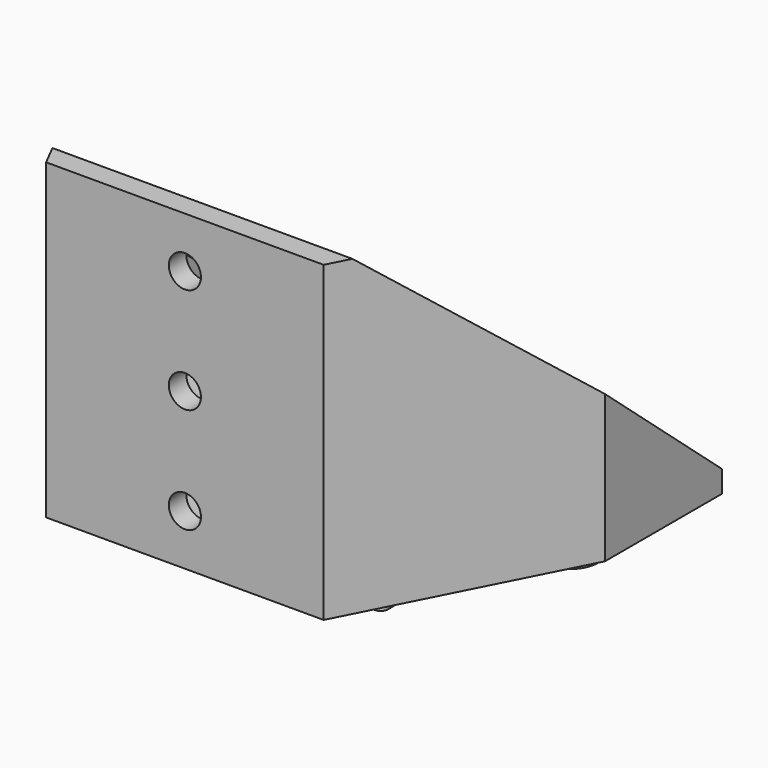
from build123d import *

# Parameters (mm, degrees)
F4_DEPTH       = 21.4
F5_DEPTH       = 1.5
F1_R           = 1.9
F1_W           = 19
F1_H           = 1.5
F6_DEPTH       = 1.6
F8_DEPTH       = 17.001
F8_DEPTH_BACK  = 17.001
F9_R           = 1.15
F10_DEPTH      = 21.401
F10_DEPTH_BACK = 1.601
F11_R          = 1.1
F12_DEPTH      = 1.5
F13_T1_DEPTH   = 1.5
F13_T3_DEPTH   = 36.5
F14_R          = 0.5


# Not quite as in the source:
# - a fillet or chamfer that OpenCascade refuses, or shapes differently, is made with other operations: its cross-section is extruded or revolved along the edge and cut away or added


with BuildPart() as f4:
    # F3 (on face) → F4 (new body)
    with BuildSketch(Plane.XY):
        Polygon((-15.5, 10), (-17, 10), (-17, 0), (-9.5, -14.7), (0, -14.7), (9.5, -14.7), (17, 0), (17, 10), (15.5, 10), (15.5, 0.3605454095), (8.5813543829, -13.2), (0, -13.2), (-8.5813543829, -13.2), (-15.5, 0.3605454095), align=None)
    extrude(amount=F4_DEPTH)

    # F2 (on Top) → F5 (join)
    with BuildSketch(Plane.XY):
        Polygon((-17, 0), (-9.5, -14.7), (0, -14.7), (9.5, -14.7), (17, 0), (17, 10), (10, 10), (10, -4.1), (0, -4.1), (-10, -4.1), (-10, 10), (-17, 10), align=None)
    extrude(amount=F5_DEPTH)

    # F1 (on Top) → F6 (join)
    with BuildSketch(Plane.XY):
        with Locations((-13, 2)):
            Circle(F1_R)
        with Locations((13, 2)):
            Circle(F1_R)
        with Locations((0, -8.95)):
            Rectangle(F1_W, F1_H)
    extrude(amount=-F6_DEPTH)

    # F7 (on Right) → F8 (cut, two sides)
    with BuildSketch(Plane.YZ) as f8_sk:
        Polygon((-13.2, 21.4), (10, 1.5), (10, 21.4), align=None)
    extrude(amount=-F8_DEPTH, mode=Mode.SUBTRACT)
    extrude(f8_sk.sketch, amount=F8_DEPTH_BACK, mode=Mode.SUBTRACT)

    # F9 (on Top) → F10 (cut, two sides)
    with BuildSketch(Plane.XY) as f10_sk:
        with Locations((13, 2)):
            Circle(F9_R)
        with Locations((-13, 2)):
            Circle(F9_R)
    extrude(amount=F10_DEPTH, mode=Mode.SUBTRACT)
    extrude(f10_sk.sketch, amount=-F10_DEPTH_BACK, mode=Mode.SUBTRACT)

    # F11 (on face) → F12 (cut, through all)
    with BuildSketch(Plane.XZ.offset(14.7)):
        with Locations((0, 3.475)):
            Circle(F11_R)
        with Locations((0, 17.925)):
            Circle(F11_R)
        with Locations((0, 10.7)):
            Circle(F11_R)
    extrude(amount=-F12_DEPTH, mode=Mode.SUBTRACT)

    # F13: fillet of radius 7 on 4 edges, made by hand

    # F13_s2 → F13_t1 (join)
    with BuildSketch(Plane.XY):
        with BuildLine():
            ThreePointArc((3, -4.1), (7.9497474683, -2.0497474683), (10, 2.9))
            Line((10, 2.9), (10, -4.1))
            Line((10, -4.1), (3, -4.1))
        make_face()
        with BuildLine():
            ThreePointArc((-10, 2.9), (-7.9497474683, -2.0497474683), (-3, -4.1))
            Line((-3, -4.1), (-10, -4.1))
            Line((-10, -4.1), (-10, 2.9))
        make_face()
    extrude(amount=F13_T1_DEPTH)

    # F13_s4 → F13_t3 (cut)
    with BuildSketch(Plane.XY.offset(-17.5)):
        with BuildLine():
            ThreePointArc((-17, 10), (-12.0502525317, 7.9497474683), (-10, 3))
            Line((-10, 3), (-10, 10))
            Line((-10, 10), (-17, 10))
        make_face()
        with BuildLine():
            ThreePointArc((10, 3), (12.0502525317, 7.9497474683), (17, 10))
            Line((17, 10), (10, 10))
            Line((10, 10), (10, 3))
        make_face()
    extrude(amount=F13_T3_DEPTH, mode=Mode.SUBTRACT)

    # F14
    f14_edges = [f4.edges().sort_by_distance(p)[0] for p in [
        (-9.5, -8.2, -0.8),
        (-9.5, -9.7, -0.8),
        (9.5, -8.2, -0.8),
        (9.5, -9.7, -0.8),
    ]]
    fillet(f14_edges, radius=F14_R)


solid = f4.part
